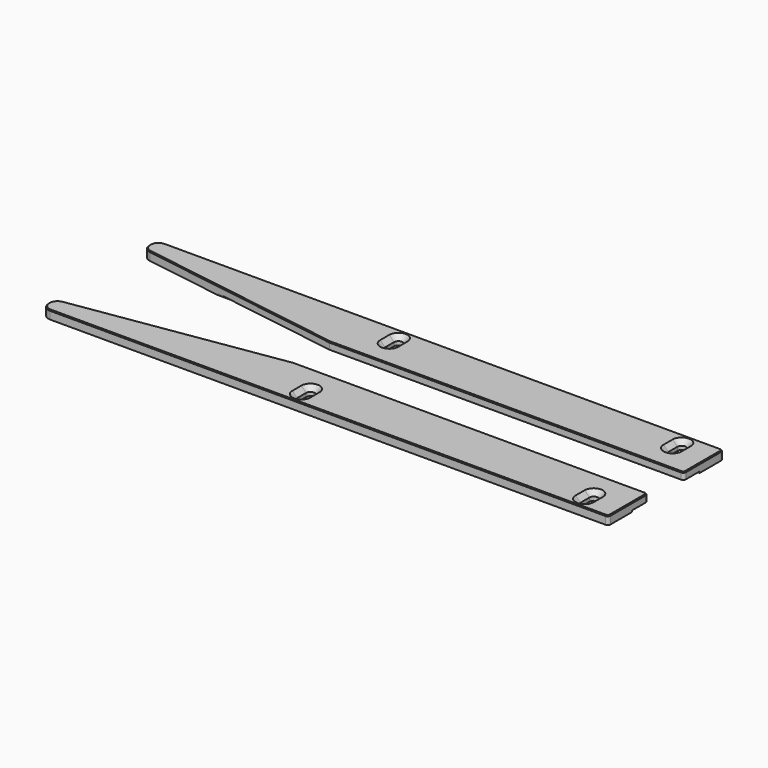
from build123d import *

# Parameters (mm, degrees)
F1_DEPTH    = 3
F2_W        = 7
F2_H        = 0.5
F3_DEPTH    = 200.001
F6_R        = 3
F6_2_R      = 3
F8_R        = 1
F8_2_R      = 1
F9_SIZE     = 0.3
F9_2_SIZE   = 0.3
F10_SIZE2   = 1.7
F10_SIZE    = 1.7
F10_2_SIZE2 = 1.7
F10_2_SIZE  = 1.7


# Not quite as in the source:
# - two fillets or chamfers of one size are made in one step
# - a feature names something its author has since deleted; it is built from what else it names


with BuildPart() as f1:
    # F0 (on Top) → F1 (new body)
    with BuildSketch(Plane.XY):
        Polygon((0, 5.8492044918), (0, 0), (200, 0), (200, 17.5), (75.0357434154, 17.5), align=None)
        with BuildLine():
            Line((89.974817574, 8), (89.974817574, 4))
            ThreePointArc((89.974817574, 4), (88.474817574, 2.5), (86.974817574, 4))
            Line((86.974817574, 4), (86.974817574, 8))
            ThreePointArc((86.974817574, 8), (88.474817574, 9.5), (89.974817574, 8))
        make_face(mode=Mode.SUBTRACT)
        with BuildLine():
            Line((189.974817574, 8), (189.974817574, 4))
            ThreePointArc((189.974817574, 4), (188.474817574, 2.5), (186.974817574, 4))
            Line((186.974817574, 4), (186.974817574, 8))
            ThreePointArc((186.974817574, 8), (188.474817574, 9.5), (189.974817574, 8))
        make_face(mode=Mode.SUBTRACT)
    extrude(amount=F1_DEPTH)

    # F2 (on face) → F3 (cut, through all)
    with BuildSketch(Plane.YZ.offset(200)):
        with Locations((14, 0.25)):
            Rectangle(F2_W, F2_H)
    extrude(amount=-F3_DEPTH, mode=Mode.SUBTRACT)


with BuildPart() as f5_1:
    # F5: instance of F1
    add(f1.part.mirror(Plane(origin=(100, 25.4, 1.5), x_dir=(1, 0, 0), z_dir=(0, -1, 0))))

    # F6#2
    f6_2_edges = [f5_1.edges().sort_by_distance(p)[0] for p in [
        (0, 44.950796, 1.5),
        (0, 50.8, 1.5),
    ]]
    fillet(f6_2_edges, radius=F6_2_R)

    # F8#2
    f8_2_edges = [f5_1.edges().sort_by_distance(p)[0] for p in [
        (200, 50.8, 1.5),
        (200, 33.3, 1.75),
    ]]
    fillet(f8_2_edges, radius=F8_2_R)

    # F9#2
    f9_2_edges = [f5_1.edges().sort_by_distance(p)[0] for p in [
        (137.017872, 33.3, 3),
        (200, 42.05, 3),
        (199.707107, 50.507107, 3),
        (101, 50.8, 3),
        (38.787725, 38.928228, 3),
        (0.87868, 49.92132, 3),
        (0.721746, 45.569124, 3),
        (0, 47.660467, 3),
        (199.707107, 33.592893, 3),
    ]]
    chamfer(f9_2_edges, length=F9_2_SIZE)

    # F10#2
    f10_2_edges = [f5_1.edges().sort_by_distance(p)[0] for p in [
        (189.974818, 44.8, 3),
        (188.474818, 41.3, 3),
        (186.974818, 44.8, 3),
        (188.474818, 48.3, 3),
        (88.474818, 48.3, 3),
        (89.974818, 44.8, 3),
        (88.474818, 41.3, 3),
        (86.974818, 44.8, 3),
    ]]
    chamfer(f10_2_edges, length=F10_2_SIZE, length2=F10_2_SIZE2)


with BuildPart() as f1_1:
    add(f1.part)

    # F6
    f6_edges = [f1_1.edges().sort_by_distance(p)[0] for p in [
        (0, 5.849204, 1.5),
        (0, 0, 1.5),
    ]]
    fillet(f6_edges, radius=F6_R)

    # F8
    f8_edges = [f1_1.edges().sort_by_distance(p)[0] for p in [
        (200, 0, 1.5),
        (200, 17.5, 1.75),
    ]]
    fillet(f8_edges, radius=F8_R)

    # F9
    f9_edges = [f1_1.edges().sort_by_distance(p)[0] for p in [
        (137.017872, 17.5, 3),
        (200, 8.75, 3),
        (199.707107, 0.292893, 3),
        (101, 0, 3),
        (38.787725, 11.871772, 3),
        (0.87868, 0.87868, 3),
        (0.721746, 5.230876, 3),
        (0, 3.139533, 3),
        (199.707107, 17.207107, 3),
    ]]
    chamfer(f9_edges, length=F9_SIZE)

    # F10
    f10_edges = [f1_1.edges().sort_by_distance(p)[0] for p in [
        (89.974818, 6, 3),
        (88.474818, 9.5, 3),
        (86.974818, 6, 3),
        (88.474818, 2.5, 3),
        (188.474818, 9.5, 3),
        (189.974818, 6, 3),
        (188.474818, 2.5, 3),
        (186.974818, 6, 3),
    ]]
    chamfer(f10_edges, length=F10_SIZE, length2=F10_SIZE2)


solid = Compound([f5_1.part, f1_1.part])
